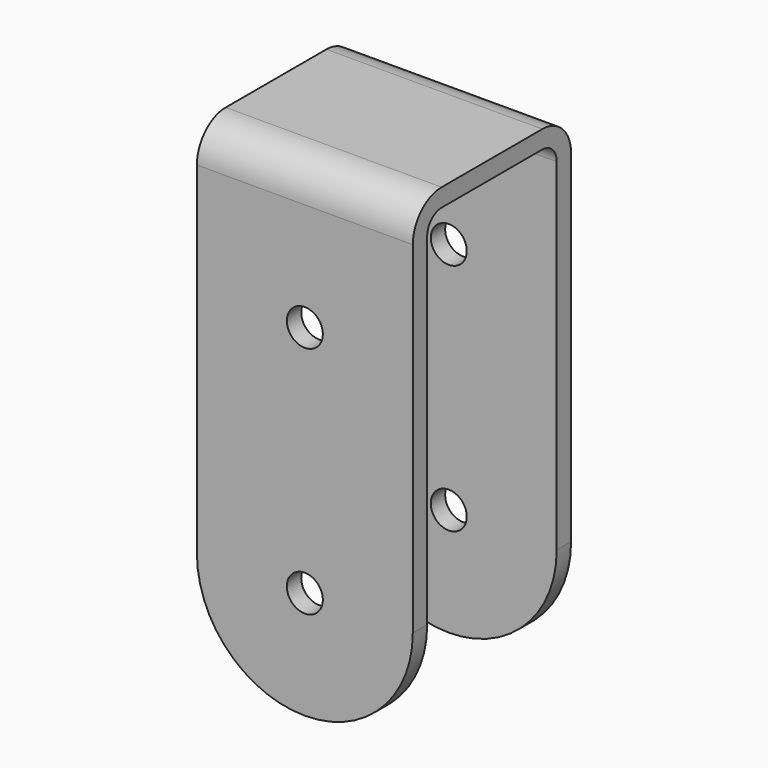
from build123d import *

# Parameters (mm, degrees)
F1_DEPTH = 38.1
F2_R     = 3.175
F3_R     = 6.35
F4_R     = 19.04999
F5_R     = 3.175
F6_DEPTH = 34.926


# Not quite as in the source:
# - a fillet or chamfer is up to 0.001 mm smaller than in the source, because OpenCascade refuses the exact size


with BuildPart() as f1:
    # F0 (on Right) → F1 (new body)
    with BuildSketch(Plane.YZ):
        Polygon((-1.5875, -4.7625), (-1.5875, 77.7875), (26.9875, 77.7875), (26.9875, -4.7625), (30.1625, -4.7625), (30.1625, 80.9625), (-4.7625, 80.9625), (-4.7625, -4.7625), align=None)
    extrude(amount=F1_DEPTH)

    # F2
    f2_edges = [f1.edges().sort_by_distance(p)[0] for p in [
        (19.05, 26.9875, 77.7875),
        (19.05, -1.5875, 77.7875),
    ]]
    fillet(f2_edges, radius=F2_R)

    # F3
    f3_edges = [f1.edges().sort_by_distance(p)[0] for p in [
        (19.05, 30.1625, 80.9625),
        (19.05, -4.7625, 80.9625),
    ]]
    fillet(f3_edges, radius=F3_R)

    # F4 (radius 19.05 in the source; OpenCascade refuses exactly that, so slightly less here)
    f4_edges = [f1.edges().sort_by_distance(p)[0] for p in [
        (38.1, 28.575, -4.7625),
        (0, 28.575, -4.7625),
        (38.1, -3.175, -4.7625),
        (0, -3.175, -4.7625),
    ]]
    fillet(f4_edges, radius=F4_R)

    # F5 (on face) → F6 (cut, through all)
    with BuildSketch(Plane(origin=(0, 30.1625, 0), x_dir=(-1, 0, 0), z_dir=(0, 1, 0))):
        with Locations((-19.05, 14.2875)):
            Circle(F5_R)
        with Locations((-19.05, 55.5625)):
            Circle(F5_R)
    extrude(amount=-F6_DEPTH, mode=Mode.SUBTRACT)


solid = f1.part
